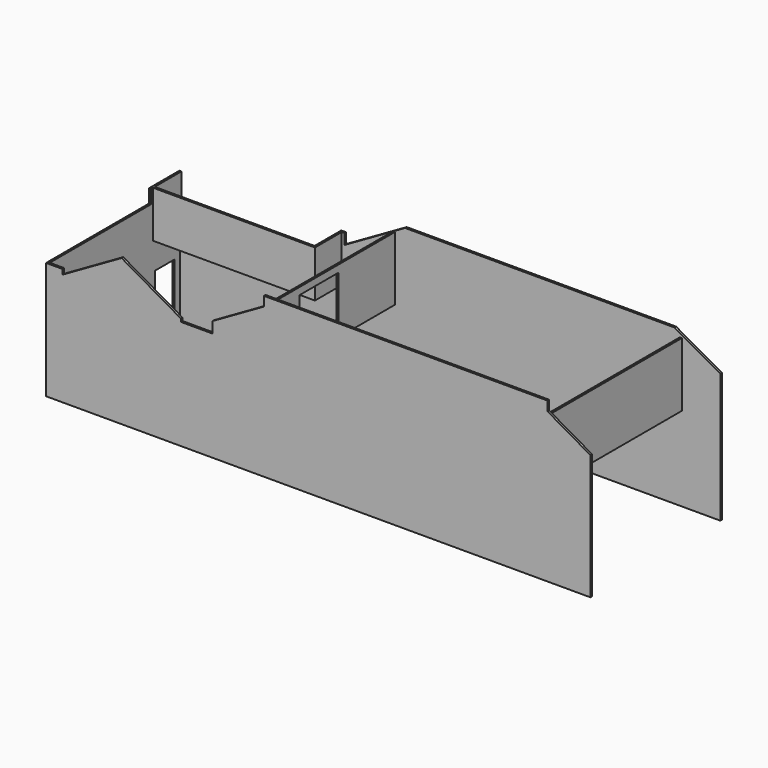
from build123d import *

# Parameters (mm, degrees)
F1_DEPTH  = 75
F3_DEPTH  = 75
F5_DEPTH  = 75
F6_W      = 1313
F6_H      = 1730
F7_DEPTH  = 75
F8_W      = 5925
F8_H      = 1730
F9_DEPTH  = 75
F11_DEPTH = 6028
F12_W     = 1822
F12_H     = 2112
F13_DEPTH = 75
F15_DEPTH = 6028


with BuildPart() as f1:
    # F0 (on Right) → F1 (new body)
    with BuildSketch(Plane.YZ):
        Polygon((0, 4352), (0, 0), (300, 0), (300, 2200), (3800, 2200), (3800, 0), (4945, 0), (4945, 2110), (5865, 2110), (5865, 0), (6178, 0), (6178, 4852), (4765, 4852), (4765, 4352), align=None)
    extrude(amount=F1_DEPTH)

    # F2 (on face) → F3 (join)
    with BuildSketch(Plane.XZ):
        Polygon((75, 4352), (75, 0), (20178, 0), (20178, 4643.0391220405), (18588, 5553.6407079484), (18588, 5903.6407079484), (8077.61993, 5903.6407079484), (8077.61993, 5553.6407079484), (6175, 4464), (6175, 4052), (5000, 4052), (5000, 4162), (2800, 5421.9518798725), (600, 4162), (600, 4352), align=None)
    extrude(amount=-F3_DEPTH)

    # F4 (on face) → F5 (join)
    with BuildSketch(Plane(origin=(0, 6178, 0), x_dir=(-1, 0, 0), z_dir=(0, 1, 0))):
        Polygon((-20113, 4798.3090141813), (-20113, 0), (-75, 0), (-75, 3122), (-6075, 3122), (-6075, 4852), (-6175, 4852), (-6175, 4464), (-8427.6199314719, 5752), (-18413.8736724854, 5752), align=None)
    extrude(amount=-F5_DEPTH)

    # F6 (on face) → F7 (join)
    with BuildSketch(Plane(origin=(6075, 0, 0), x_dir=(0, -1, 0), z_dir=(-1, 0, 0))):
        with Locations((-5521.5, 3987)):
            Rectangle(F6_W, F6_H)
    extrude(amount=F7_DEPTH)

    # F8 (on face) → F9 (join)
    with BuildSketch(Plane.XZ.offset(-4865)):
        with Locations((3037.5, 3987)):
            Rectangle(F8_W, F8_H)
    extrude(amount=-F9_DEPTH)

    # F10 (on face) → F11 (join, through all)
    with BuildSketch(Plane(origin=(0, 75, 0), x_dir=(-1, 0, 0), z_dir=(0, 1, 0))):
        Polygon((-8047.99993, 5497), (-8047.99993, 3122), (-7972.99993, 3122), (-7972.99993, 5493.7242690064), (-7978.7196787467, 5497), align=None)
    extrude(amount=F11_DEPTH)

    # F12 (on face) → F13 (cut, through all)
    with BuildSketch(Plane(origin=(7972.99993, 0, 0), x_dir=(0, -1, 0), z_dir=(-1, 0, 0))):
        with Locations((-2586, 4178)):
            Rectangle(F12_W, F12_H)
    extrude(amount=-F13_DEPTH, mode=Mode.SUBTRACT)

    # F14 (on face) → F15 (join, through all)
    with BuildSketch(Plane(origin=(0, 75, 0), x_dir=(-1, 0, 0), z_dir=(0, 1, 0))):
        Polygon((-18688, 5496.3701679542), (-18688, 3122), (-18613, 3122), (-18613, 5497), (-18686.9002512533, 5497), align=None)
    extrude(amount=F15_DEPTH)


solid = f1.part
